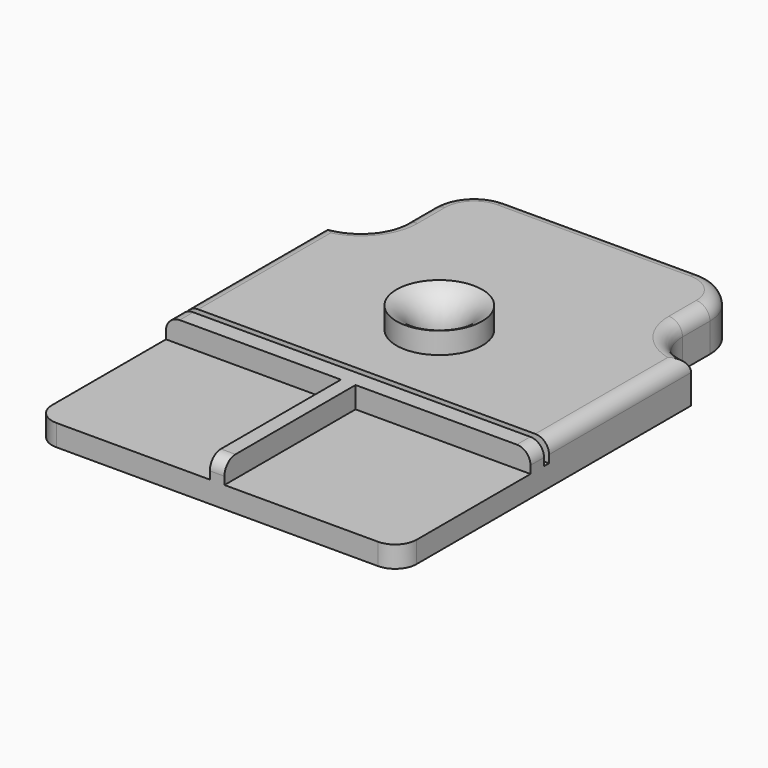
from build123d import *

# Parameters (mm, degrees)
F1_DEPTH  = 3.175
F2_R      = 1.016
F3_W      = 24.9555
F3_H      = 0.4668365944
F3_W_2    = 8.3583763037
F3_W_3    = 6.5895795759
F4_DEPTH  = 1.5875
F5_R      = 1.524
F6_DEPTH  = 25.4
F5_R_2    = 3.175
F7_DEPTH  = 1.5875
F9_W      = 1.294683665
F9_H      = 1.482822001
F10_DEPTH = 2.8222222222
F11_R     = 0.79375
F12_DEPTH = 5.08
F13_R     = 0.254
F15_DEPTH = 2.8222222222


# Not quite as in the source:
# - a fillet or chamfer that OpenCascade refuses, or shapes differently, is made with other operations: its cross-section is extruded or revolved along the edge and cut away or added


with BuildPart() as f1:
    # F0 (on Top) → F1 (new body)
    with BuildSketch(Plane.XY):
        with BuildLine():
            ThreePointArc((0, 1.5875), (0.4649679849, 0.4649679849), (1.5875, 0))
            Line((1.5875, 0), (25.4, 0))
            ThreePointArc((25.4, 0), (26.5225320151, 0.4649679849), (26.9875, 1.5875))
            Line((26.9875, 1.5875), (26.9875, 26.9875))
            ThreePointArc((26.9875, 26.9875), (24.7424359697, 27.9174359697), (23.8125, 30.1625))
            Line((23.8125, 30.1625), (23.8125, 32.7025))
            ThreePointArc((23.8125, 32.7025), (22.8825640303, 34.9475640303), (20.6375, 35.8775))
            Line((20.6375, 35.8775), (6.35, 35.8775))
            ThreePointArc((6.35, 35.8775), (4.1049359697, 34.9475640303), (3.175, 32.7025))
            Line((3.175, 32.7025), (3.175, 30.1625))
            ThreePointArc((3.175, 30.1625), (2.2450640303, 27.9174359697), (0, 26.9875))
            Line((0, 26.9875), (0, 1.5875))
        make_face()
    extrude(amount=F1_DEPTH)

    # F2
    f2_edges = [f1.edges().sort_by_distance(p)[0] for p in [
        (26.9875, 14.2875, 3.175),
        (3.175, 31.4325, 3.175),
        (2.245064, 27.917436, 3.175),
        (24.742436, 27.917436, 3.175),
        (23.8125, 31.4325, 3.175),
        (22.882564, 34.947564, 3.175),
        (13.49375, 35.8775, 3.175),
        (4.104936, 34.947564, 3.175),
    ]]
    fillet(f2_edges, radius=F2_R)

    # F3 (on face) → F4 (cut)
    with BuildSketch(Plane.XY.offset(3.175)):
        with BuildLine():
            Line((43.3063970949, 12.1285), (25.9715, 12.1285))
            Line((25.9715, 12.1285), (25.9715, 1.5875))
            ThreePointArc((25.9715, 1.5875), (25.8041115254, 1.1833884746), (25.4, 1.016))
            Line((25.4, 1.016), (14.0335, 1.016))
            Line((14.0335, 1.016), (14.0335, -10.401187452))
            Line((14.0335, -10.401187452), (43.3063970949, -10.401187452))
            Line((43.3063970949, -10.401187452), (43.3063970949, 12.1285))
        make_face()
        with BuildLine():
            Line((25.9715, 12.1285), (14.0335, 12.1285))
            Line((14.0335, 12.1285), (14.0335, 1.016))
            Line((14.0335, 1.016), (25.4, 1.016))
            ThreePointArc((25.4, 1.016), (25.8041115254, 1.1833884746), (25.9715, 1.5875))
            Line((25.9715, 1.5875), (25.9715, 12.1285))
        make_face()
        with BuildLine():
            Line((1.5875, 1.016), (12.954, 1.016))
            Line((12.954, 1.016), (12.954, 12.1285))
            Line((12.954, 12.1285), (1.016, 12.1285))
            Line((1.016, 12.1285), (1.016, 1.5875))
            ThreePointArc((1.016, 1.5875), (1.1833884746, 1.1833884746), (1.5875, 1.016))
        make_face()
        with BuildLine():
            Line((12.954, -10.9148975462), (12.954, 1.016))
            Line((12.954, 1.016), (1.5875, 1.016))
            ThreePointArc((1.5875, 1.016), (1.1833884746, 1.1833884746), (1.016, 1.5875))
            Line((1.016, 1.5875), (1.016, 12.1285))
            Line((1.016, 12.1285), (-5.5735795759, 12.1285))
            Line((-5.5735795759, 12.1285), (-5.5735795759, -10.9148975462))
            Line((-5.5735795759, -10.9148975462), (12.954, -10.9148975462))
        make_face()
        with Locations((13.49375, 13.6085897574)):
            Rectangle(F3_W, F3_H)
        with Locations((30.1506881518, 13.6085897574)):
            Rectangle(F3_W_2, F3_H)
        with Locations((-2.2787897879, 13.6085897574)):
            Rectangle(F3_W_3, F3_H)
    extrude(amount=-F4_DEPTH, mode=Mode.SUBTRACT)

    # F5 (on face) → F6 (cut)
    with BuildSketch(Plane.XY.offset(3.175)):
        with Locations((13.49375, 20.5581425011)):
            Circle(F5_R)
    extrude(amount=-F6_DEPTH, mode=Mode.SUBTRACT)

    # F5 (on face) → F7 (join)
    with BuildSketch(Plane.XY.offset(3.175)):
        with Locations((13.49375, 20.5581425011)):
            Circle(F5_R_2)
        with Locations((13.49375, 20.5581425011)):
            Circle(F5_R, mode=Mode.SUBTRACT)
    extrude(amount=F7_DEPTH)

    # F8: fillet of radius 2.54 on 1 edges, made by hand

    # F8_s1 → F8_t2 (revolve, cut)
    with BuildSketch(Plane.XZ.offset(-20.5581425011)):
        with BuildLine():
            ThreePointArc((15.01775, 2.3831557626), (15.4709270559, 3.8311785525), (16.66875, 4.7625))
            Line((16.66875, 4.7625), (15.01775, 4.7625))
            Line((15.01775, 4.7625), (15.01775, 2.3831557626))
        make_face()
    revolve(axis=Axis((13.49375, 20.5581425011, 4.7625), (0, 0, 1)), mode=Mode.SUBTRACT)

    # F9 (on face) → F10 (cut)
    with BuildSketch(Plane(origin=(0, 0, 0), x_dir=(1, 0, 0), z_dir=(0, 0, -1))):
        with BuildLine():
            ThreePointArc((15.1753826067, -15.5802866697), (17.8362583784, -17.462592513), (18.8565061088, -20.5581425011))
            Line((18.8565061088, -20.5581425011), (26.1830221862, -20.5581425011))
            Line((26.1830221862, -20.5581425011), (26.1830221862, -15.5802866697))
            Line((26.1830221862, -15.5802866697), (15.1753826067, -15.5802866697))
        make_face()
        with BuildLine():
            Line((26.1830221862, -20.5581425011), (18.8565061088, -20.5581425011))
            ThreePointArc((18.8565061088, -20.5581425011), (17.8362583784, -23.6536924892), (15.1753826067, -25.5359983325))
            Line((15.1753826067, -25.5359983325), (24.8883385211, -25.5359983325))
            Line((24.8883385211, -25.5359983325), (24.8883385211, -24.0531763315))
            Line((24.8883385211, -24.0531763315), (26.1830221862, -24.0531763315))
            Line((26.1830221862, -24.0531763315), (26.1830221862, -20.5581425011))
        make_face()
        with Locations((25.5356803536, -24.794587332)):
            Rectangle(F9_W, F9_H)
        with BuildLine():
            Line((12.1251240555, -15.5802866697), (1.117484476, -15.5802866697))
            Line((1.117484476, -15.5802866697), (1.117484476, -20.5581425011))
            Line((1.117484476, -20.5581425011), (1.117484476, -25.5359983325))
            Line((1.117484476, -25.5359983325), (12.1251240555, -25.5359983325))
            ThreePointArc((12.1251240555, -25.5359983325), (8.4440005534, -20.5581425011), (12.1251240555, -15.5802866697))
        make_face()
    extrude(amount=-F10_DEPTH, mode=Mode.SUBTRACT)

    # F11 (on face) → F12 (join)
    with BuildSketch(Plane(origin=(0, 0, 2.8222222222), x_dir=(1, 0, 0), z_dir=(0, 0, -1))):
        with Locations((22.4790647626, -20.5581425011)):
            Circle(F11_R)
        with Locations((4.8214418996, -21.3518925011)):
            Circle(F11_R)
    extrude(amount=F12_DEPTH)

    # F13
    f13_edges = [f1.edges().sort_by_distance(p)[0] for p in [
        (21.685315, 20.558143, -2.257778),
        (4.027692, 21.351893, -2.257778),
    ]]
    fillet(f13_edges, radius=F13_R)

    # F14 (on face) → F15 (cut)
    with BuildSketch(Plane(origin=(0, 0, 0), x_dir=(1, 0, 0), z_dir=(0, 0, -1))):
        with BuildLine():
            Line((10.4354891836, -27.7508334085), (3.8518141955, -27.7508334085))
            Line((3.8518141955, -27.7508334085), (3.8518141955, -29.2588919401))
            ThreePointArc((3.8518141955, -29.2588919401), (7.5132373167, -33.3483248509), (12.7214891836, -35.0814126432))
            Line((12.7214891836, -35.0814126432), (12.7214891836, -30.0368334085))
            ThreePointArc((12.7214891836, -30.0368334085), (12.0519352854, -28.4203873067), (10.4354891836, -27.7508334085))
        make_face()
        with BuildLine():
            ThreePointArc((14.0368680542, -35.0814126432), (19.2451199211, -33.3483248509), (22.9065430423, -29.2588919401))
            Line((22.9065430423, -29.2588919401), (22.9065430423, -27.7508334085))
            Line((22.9065430423, -27.7508334085), (16.3228680542, -27.7508334085))
            ThreePointArc((16.3228680542, -27.7508334085), (14.7064219524, -28.4203873067), (14.0368680542, -30.0368334085))
            Line((14.0368680542, -30.0368334085), (14.0368680542, -35.0814126432))
        make_face()
    extrude(amount=-F15_DEPTH, mode=Mode.SUBTRACT)


solid = f1.part
